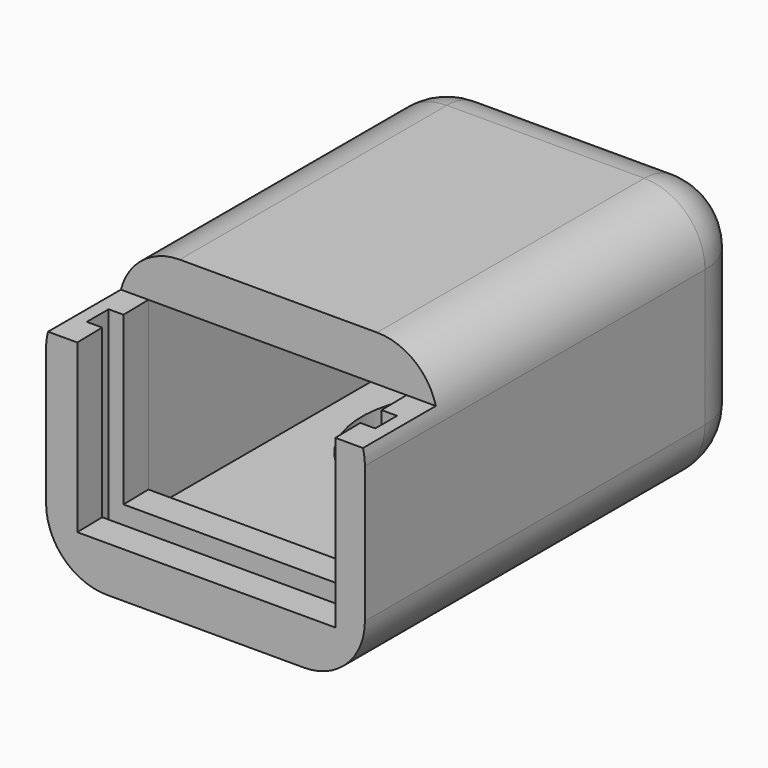
from build123d import *

# Parameters (mm, degrees)
F0_W     = 8.5
F0_H     = 11.400557369
F0_W_2   = 0.9711329822
F0_H_2   = 1.599442631
F0_W_3   = 1.0288670178
F1_DEPTH = 0.9
F2_DEPTH = 1.5
F3_DEPTH = 7
F5_W     = 10.5
F5_H     = 13
F6_DEPTH = 1.5
F7_R     = 2
F9_DEPTH = 0.9


# Not quite as in the source:
# - a feature names something its author has since deleted; it is built from what else it names


with BuildPart() as f1:
    # F0 (on Top) → F1 (new body)
    with BuildSketch(Plane.XY):
        with Locations((-0.0288670178, 7.2002786845)):
            Rectangle(F0_W, F0_H)
        Polygon((-5.25, 1.5), (-5.25, -1.5), (-4.2211329822, -1.5), (-4.2413398946, -0.45), (-4.75, -0.45), (-4.75, 0.45), (-4.2586601054, 0.45), (-4.2788670178, 1.5), align=None)
        Polygon((4.2211329822, 1.5), (-4.2788670178, 1.5), (-4.2586601054, 0.45), (4.2413398946, 0.45), align=None)
        with Locations((-4.7644335089, 7.2002786845)):
            Rectangle(F0_W_2, F0_H)
        Polygon((4.2586601054, -0.45), (4.2788670178, -1.5), (5.25, -1.5), (5.25, 1.5), (4.2211329822, 1.5), (4.2413398946, 0.45), (4.75, 0.45), (4.75, -0.45), align=None)
        Polygon((-4.2413398946, -0.45), (-4.2211329822, -1.5), (4.2788670178, -1.5), (4.2586601054, -0.45), align=None)
        Polygon((-4.2586601054, 0.45), (-4.2413398946, -0.45), (4.2586601054, -0.45), (4.2413398946, 0.45), align=None)
        Polygon((-4.75, -0.45), (-4.2413398946, -0.45), (-4.2586601054, 0.45), (-4.75, 0.45), align=None)
        Polygon((4.2413398946, 0.45), (4.2586601054, -0.45), (4.75, -0.45), (4.75, 0.45), align=None)
        with Locations((-4.7644335089, 13.7002786845)):
            Rectangle(F0_W_2, F0_H_2)
        with Locations((-0.0288670178, 13.7002786845)):
            Rectangle(F0_W, F0_H_2)
        with Locations((4.7355664911, 13.7002786845)):
            Rectangle(F0_W_3, F0_H_2)
        with Locations((4.7355664911, 7.2002786845)):
            Rectangle(F0_W_3, F0_H)
    extrude(amount=F1_DEPTH)

    # F0 (on Top) → F2 (join)
    with BuildSketch(Plane.XY):
        Polygon((-4.2413398946, -0.45), (-4.2211329822, -1.5), (4.2788670178, -1.5), (4.2586601054, -0.45), align=None)
        Polygon((-5.25, 1.5), (-5.25, -1.5), (-4.2211329822, -1.5), (-4.2413398946, -0.45), (-4.75, -0.45), (-4.75, 0.45), (-4.2586601054, 0.45), (-4.2788670178, 1.5), align=None)
        Polygon((4.2586601054, -0.45), (4.2788670178, -1.5), (5.25, -1.5), (5.25, 1.5), (4.2211329822, 1.5), (4.2413398946, 0.45), (4.75, 0.45), (4.75, -0.45), align=None)
        Polygon((4.2211329822, 1.5), (-4.2788670178, 1.5), (-4.2586601054, 0.45), (4.2413398946, 0.45), align=None)
        with Locations((-4.7644335089, 7.2002786845)):
            Rectangle(F0_W_2, F0_H)
        with Locations((-4.7644335089, 13.7002786845)):
            Rectangle(F0_W_2, F0_H_2)
        with Locations((-0.0288670178, 13.7002786845)):
            Rectangle(F0_W, F0_H_2)
        with Locations((4.7355664911, 13.7002786845)):
            Rectangle(F0_W_3, F0_H_2)
        with Locations((4.7355664911, 7.2002786845)):
            Rectangle(F0_W_3, F0_H)
    extrude(amount=F2_DEPTH)

    # F0 (on Top) → F3 (join)
    with BuildSketch(Plane.XY):
        Polygon((-5.25, 1.5), (-5.25, -1.5), (-4.2211329822, -1.5), (-4.2413398946, -0.45), (-4.75, -0.45), (-4.75, 0.45), (-4.2586601054, 0.45), (-4.2788670178, 1.5), align=None)
        Polygon((4.2586601054, -0.45), (4.2788670178, -1.5), (5.25, -1.5), (5.25, 1.5), (4.2211329822, 1.5), (4.2413398946, 0.45), (4.75, 0.45), (4.75, -0.45), align=None)
        with Locations((-4.7644335089, 13.7002786845)):
            Rectangle(F0_W_2, F0_H_2)
        with Locations((-0.0288670178, 13.7002786845)):
            Rectangle(F0_W, F0_H_2)
        with Locations((4.7355664911, 13.7002786845)):
            Rectangle(F0_W_3, F0_H_2)
        with Locations((-4.7644335089, 7.2002786845)):
            Rectangle(F0_W_2, F0_H)
        with Locations((4.7355664911, 7.2002786845)):
            Rectangle(F0_W_3, F0_H)
    extrude(amount=F3_DEPTH)

    # F5 (on offset) → F6 (join)
    with BuildSketch(Plane.XY.offset(7)):
        with Locations((0, 8)):
            Rectangle(F5_W, F5_H)
    extrude(amount=F6_DEPTH)

    # F7
    f7_edges = [f1.edges().sort_by_distance(p)[0] for p in [
        (5.25, 14.5, 4.25),
        (0, 14.5, 8.5),
        (5.25, 8, 8.5),
        (5.25, 6.5, 0),
        (0, 14.5, 0),
        (-5.25, 6.5, 0),
        (-5.25, 14.5, 4.25),
        (-5.25, 8, 8.5),
    ]]
    fillet(f7_edges, radius=F7_R)

    # F8 (on Top) → F9 (cut, through all)
    with BuildSketch(Plane.XY):
        with BuildLine():
            ThreePointArc((0, 5.75), (2.2980970389, 6.7019029611), (3.25, 9))
            ThreePointArc((3.25, 9), (-2.2980970389, 11.2980970389), (0, 5.75))
        make_face()
    extrude(amount=F9_DEPTH, mode=Mode.SUBTRACT)


solid = f1.part
